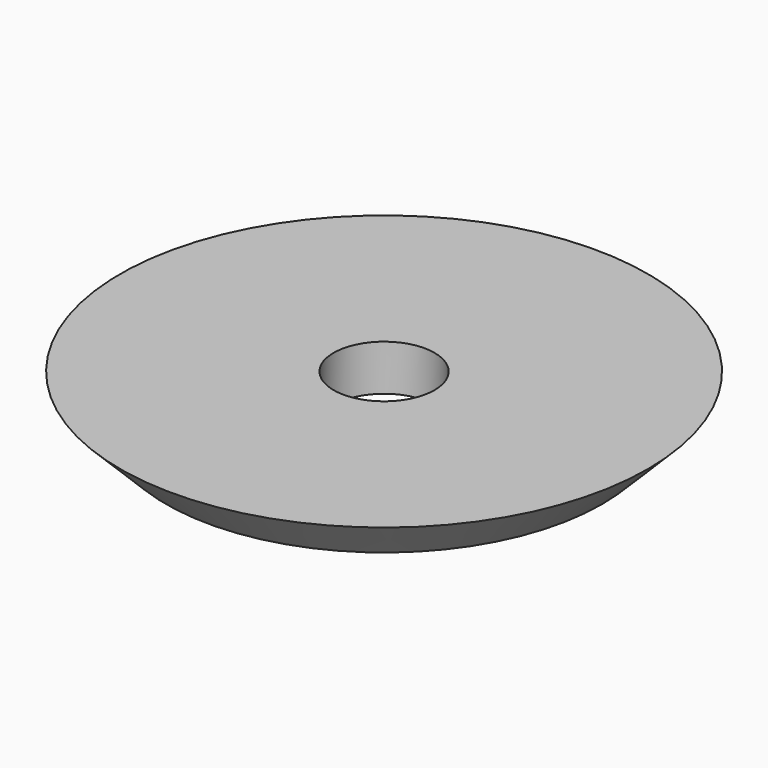
from build123d import *

# Parameters (mm, degrees)
F0_R     = 29.21
F0_R_2   = 5.588
F1_DEPTH = 5.08
F2_SIZE  = 5.07999


# Not quite as in the source:
# - a fillet or chamfer is up to 0.001 mm smaller than in the source, because OpenCascade refuses the exact size


with BuildPart() as f1:
    # F0 (on Top) → F1 (new body)
    with BuildSketch(Plane.XY):
        Circle(F0_R)
        Circle(F0_R_2, mode=Mode.SUBTRACT)
    extrude(amount=F1_DEPTH)

    # F2 (size 5.08 in the source; OpenCascade refuses exactly that, so slightly less here)
    f2_edges = [f1.edges().sort_by_distance(p)[0] for p in [
        (-29.21, 0, 0),
    ]]
    chamfer(f2_edges, length=F2_SIZE)


solid = f1.part
